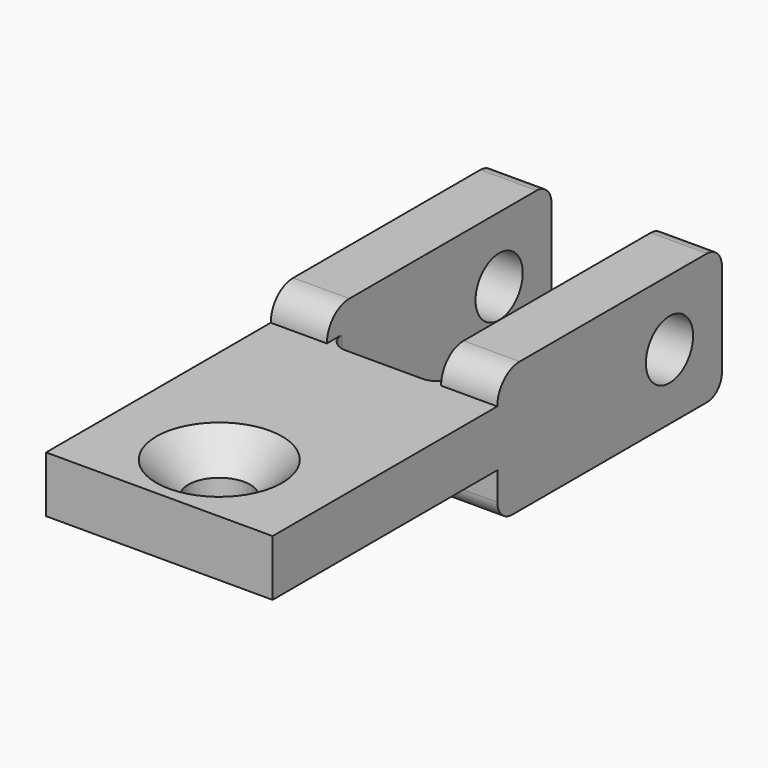
from build123d import *

# Parameters (mm, degrees)
F0_W           = 3.05
F0_H           = 15
F1_DEPTH       = 3
F3_DEPTH       = 3
F6_D           = 3.3
F6_CSINK_D     = 6.72
F6_CSINK_ANGLE = 90
F8_D           = 3.15
F9_T1_DEPTH    = 3
F9_T3_DEPTH    = 8
F9_T5_DEPTH    = 8


# Not quite as in the source:
# - a fillet or chamfer that OpenCascade refuses, or shapes differently, is made with other operations: its cross-section is extruded or revolved along the edge and cut away or added


with BuildPart() as f1:
    # F0 (on Top) → F1 (new body)
    with BuildSketch(Plane.XY):
        with Locations((1.525, 7.5)):
            Rectangle(F0_W, F0_H)
    extrude(amount=F1_DEPTH)

    # F2 (on face) → F3 (join)
    with BuildSketch(Plane.YZ.offset(3.05)):
        with BuildLine():
            Line((0, 3), (0, 0))
            Line((0, 0), (15, 0))
            Line((15, 0), (15, -2.5))
            Line((15, -2.5), (30, -2.5))
            Line((30, -2.5), (30, 4.5))
            Line((30, 4.5), (16.5, 4.5))
            ThreePointArc((16.5, 4.5), (15.4393398282, 4.0606601718), (15, 3))
            Line((15, 3), (0, 3))
        make_face()
    extrude(amount=F3_DEPTH)

    # F4: F1 across face


with BuildPart() as f1_1:
    add(f1.part)
    add(f1.part.mirror(Plane(origin=(0, 7.5, 1.5), x_dir=(0, -1, 0), z_dir=(-1, 0, 0))))

    # F6 (through all)
    with Locations(Plane.XY.offset(3)):
        with Locations((0, 4)):
            CounterSinkHole(F6_D / 2, F6_CSINK_D / 2, counter_sink_angle=F6_CSINK_ANGLE)

    # F8 (through all)
    with Locations(Plane.YZ.offset(6.05)):
        with Locations((26.5, 1)):
            Hole(F8_D / 2)

    # F9: fillet of radius 1 on 8 edges, made by hand

    # F9_s2 → F9_t1 (join)
    with BuildSketch(Plane.XY):
        with BuildLine():
            ThreePointArc((2.05, 15), (2.7571067812, 15.2928932188), (3.05, 16))
            Line((3.05, 16), (3.05, 15))
            Line((3.05, 15), (2.05, 15))
        make_face()
        with BuildLine():
            ThreePointArc((-2.05, 15), (-2.7571067812, 15.2928932188), (-3.05, 16))
            Line((-3.05, 16), (-3.05, 15))
            Line((-3.05, 15), (-2.05, 15))
        make_face()
    extrude(amount=F9_T1_DEPTH)

    # F9_s4 → F9_t3 (cut)
    with BuildSketch(Plane.YZ.offset(0.55)):
        with BuildLine():
            ThreePointArc((29, 4.5), (29.7071067812, 4.2071067812), (30, 3.5))
            Line((30, 3.5), (30, 4.5))
            Line((30, 4.5), (29, 4.5))
        make_face()
        with BuildLine():
            ThreePointArc((29, -2.5), (29.7071067812, -2.2071067812), (30, -1.5))
            Line((30, -1.5), (30, -2.5))
            Line((30, -2.5), (29, -2.5))
        make_face()
        with BuildLine():
            ThreePointArc((15, -1.5), (15.2928932188, -2.2071067812), (16, -2.5))
            Line((16, -2.5), (15, -2.5))
            Line((15, -2.5), (15, -1.5))
        make_face()
    extrude(amount=F9_T3_DEPTH, mode=Mode.SUBTRACT)

    # F9_s6 → F9_t5 (cut)
    with BuildSketch(Plane.YZ.offset(-8.55)):
        with BuildLine():
            ThreePointArc((29, 4.5), (29.7071067812, 4.2071067812), (30, 3.5))
            Line((30, 3.5), (30, 4.5))
            Line((30, 4.5), (29, 4.5))
        make_face()
        with BuildLine():
            ThreePointArc((29, -2.5), (29.7071067812, -2.2071067812), (30, -1.5))
            Line((30, -1.5), (30, -2.5))
            Line((30, -2.5), (29, -2.5))
        make_face()
        with BuildLine():
            ThreePointArc((15, -1.5), (15.2928932188, -2.2071067812), (16, -2.5))
            Line((16, -2.5), (15, -2.5))
            Line((15, -2.5), (15, -1.5))
        make_face()
    extrude(amount=F9_T5_DEPTH, mode=Mode.SUBTRACT)


solid = f1_1.part
